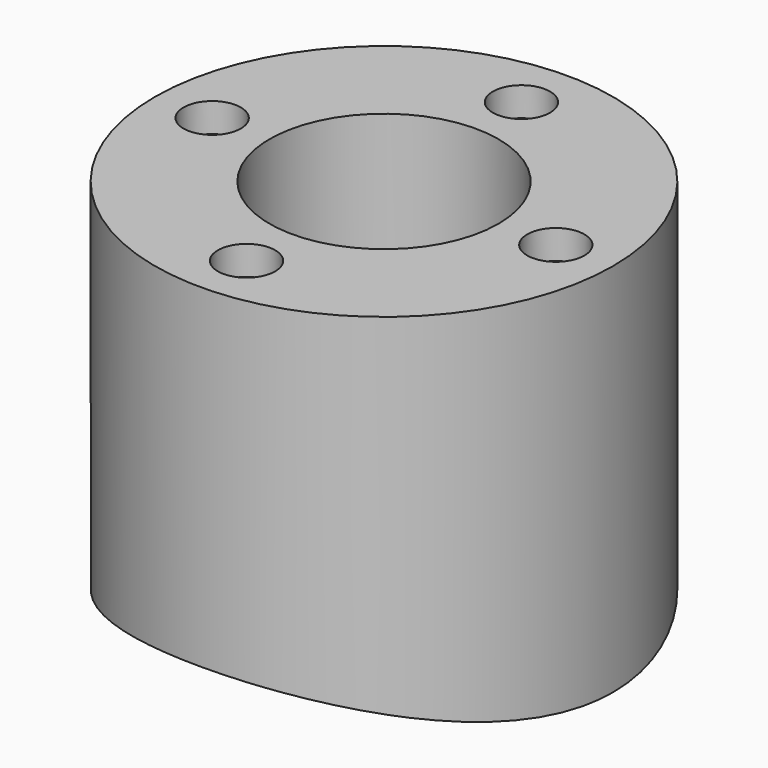
from build123d import *

# Parameters (mm, degrees)
F0_R            = 38.1
F0_R_2          = 19.05
F1_DEPTH        = 63.5
F3_COPIES_COUNT = 4
F4_R            = 109.5375
F5_DEPTH        = 38.101
F5_DEPTH_BACK   = 38.101


# Not quite as in the source:
# - a pattern or mirror of a feature is missing from the dataset's text; its kind, count and spacing are read off the source's solid


with BuildPart() as f1:
    # F0 (on Top) → F1 (new body)
    with BuildSketch(Plane.XY):
        Circle(F0_R)
        Circle(F0_R_2, mode=Mode.SUBTRACT)
    extrude(amount=F1_DEPTH)

    # F2 (on Front) → F3 (revolve, cut)
    with BuildSketch(Plane.XZ):
        Polygon((28.575, 0), (28.575, 63.5), (23.8125, 63.5), (23.8125, 58.674), (25.7683, 58.674), (25.7683, 0), align=None)
    f3 = revolve(axis=Axis((28.575, 0, 28.6447224574), (0, 0, -1)), mode=Mode.SUBTRACT)

    # F3_copies: F3 ×4 about axis
    f3_copies_axis = Axis((0, 0, 0), (0, 0, 1))
    for i in range(1, F3_COPIES_COUNT):
        add(f3.rotate(f3_copies_axis, i * 360 / F3_COPIES_COUNT), mode=Mode.SUBTRACT)

    # F4 (on Front) → F5 (cut, two sides)
    with BuildSketch(Plane.XZ) as f5_sk:
        with Locations((0, -101.6)):
            Circle(F4_R)
    extrude(amount=-F5_DEPTH, mode=Mode.SUBTRACT)
    extrude(f5_sk.sketch, amount=F5_DEPTH_BACK, mode=Mode.SUBTRACT)


solid = f1.part
